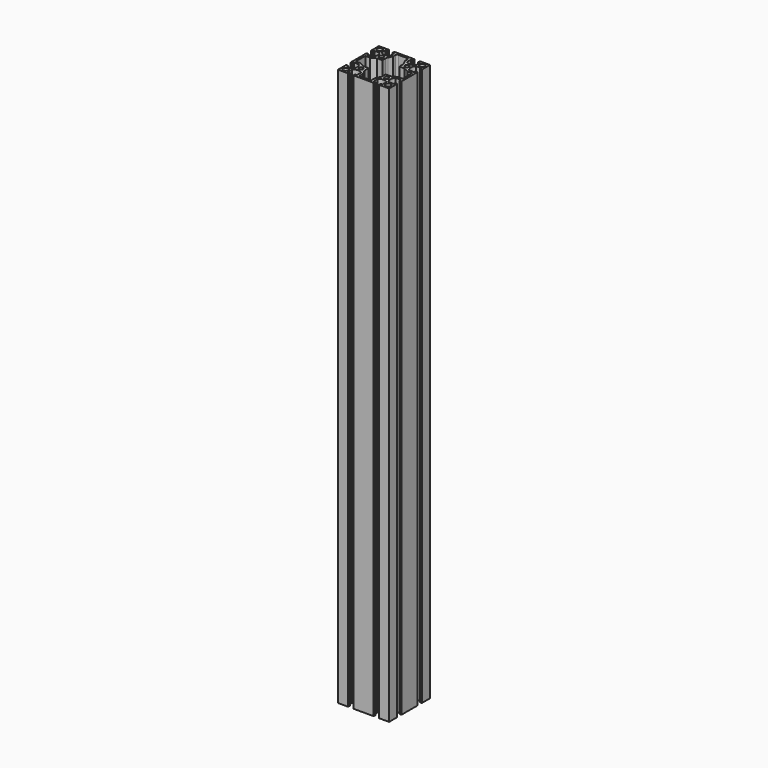
from build123d import *

# Parameters (mm, degrees)
F0_R     = 3
F0_R_2   = 2.5
F1_DEPTH = 655
F2_R     = 2
F3_R     = 7


# Not quite as in the source:
# - a feature names something its author has since deleted; it is built from what else it names


with BuildPart() as f1:
    # F0 (on Top) → F1 (new body)
    with BuildSketch(Plane.XY):
        with BuildLine():
            Line((18.15, -30), (30, -30))
            Line((30, -30), (30, -18.15))
            Line((30, -18.15), (27.5, -18.15))
            Line((27.5, -18.15), (27.5, -20.15))
            Line((27.5, -20.15), (21.5477069044, -20.15))
            ThreePointArc((21.5477069044, -20.15), (19.5, -15), (21.5477069044, -9.85))
            Line((21.5477069044, -9.85), (27.5, -9.85))
            Line((27.5, -9.85), (27.5, -11.85))
            Line((27.5, -11.85), (30, -11.85))
            Line((30, -11.85), (30, 11.85))
            Line((30, 11.85), (27.5, 11.85))
            Line((27.5, 11.85), (27.5, 9.85))
            Line((27.5, 9.85), (21.5477069044, 9.85))
            ThreePointArc((21.5477069044, 9.85), (19.5, 15), (21.5477069044, 20.15))
            Line((21.5477069044, 20.15), (27.5, 20.15))
            Line((27.5, 20.15), (27.5, 18.15))
            Line((27.5, 18.15), (30, 18.15))
            Line((30, 18.15), (30, 30))
            Line((30, 30), (18.15, 30))
            Line((18.15, 30), (18.15, 27.5))
            Line((18.15, 27.5), (20.15, 27.5))
            Line((20.15, 27.5), (20.15, 21.5477069044))
            ThreePointArc((20.15, 21.5477069044), (15, 19.5), (9.85, 21.5477069044))
            Line((9.85, 21.5477069044), (9.85, 27.5))
            Line((9.85, 27.5), (11.85, 27.5))
            Line((11.85, 27.5), (11.85, 30))
            Line((11.85, 30), (-11.85, 30))
            Line((-11.85, 30), (-11.85, 27.5))
            Line((-11.85, 27.5), (-9.85, 27.5))
            Line((-9.85, 27.5), (-9.85, 21.5477069044))
            ThreePointArc((-9.85, 21.5477069044), (-15, 19.5), (-20.15, 21.5477069044))
            Line((-20.15, 21.5477069044), (-20.15, 27.5))
            Line((-20.15, 27.5), (-18.15, 27.5))
            Line((-18.15, 27.5), (-18.15, 30))
            Line((-18.15, 30), (-30, 30))
            Line((-30, 30), (-30, 18.15))
            Line((-30, 18.15), (-27.5, 18.15))
            Line((-27.5, 18.15), (-27.5, 20.15))
            Line((-27.5, 20.15), (-21.5477069044, 20.15))
            ThreePointArc((-21.5477069044, 20.15), (-19.5, 15), (-21.5477069044, 9.85))
            Line((-21.5477069044, 9.85), (-27.5, 9.85))
            Line((-27.5, 9.85), (-27.5, 11.85))
            Line((-27.5, 11.85), (-30, 11.85))
            Line((-30, 11.85), (-30, -11.85))
            Line((-30, -11.85), (-27.5, -11.85))
            Line((-27.5, -11.85), (-27.5, -9.85))
            Line((-27.5, -9.85), (-21.5477069044, -9.85))
            ThreePointArc((-21.5477069044, -9.85), (-19.5, -15), (-21.5477069044, -20.15))
            Line((-21.5477069044, -20.15), (-27.5, -20.15))
            Line((-27.5, -20.15), (-27.5, -18.15))
            Line((-27.5, -18.15), (-30, -18.15))
            Line((-30, -18.15), (-30, -30))
            Line((-30, -30), (-18.15, -30))
            Line((-18.15, -30), (-18.15, -27.5))
            Line((-18.15, -27.5), (-20.15, -27.5))
            Line((-20.15, -27.5), (-20.15, -21.5477069044))
            ThreePointArc((-20.15, -21.5477069044), (-15, -19.5), (-9.85, -21.5477069044))
            Line((-9.85, -21.5477069044), (-9.85, -27.5))
            Line((-9.85, -27.5), (-11.85, -27.5))
            Line((-11.85, -27.5), (-11.85, -30))
            Line((-11.85, -30), (11.85, -30))
            Line((11.85, -30), (11.85, -27.5))
            Line((11.85, -27.5), (9.85, -27.5))
            Line((9.85, -27.5), (9.85, -21.5477069044))
            ThreePointArc((9.85, -21.5477069044), (15, -19.5), (20.15, -21.5477069044))
            Line((20.15, -21.5477069044), (20.15, -27.5))
            Line((20.15, -27.5), (18.15, -27.5))
            Line((18.15, -27.5), (18.15, -30))
        make_face()
        with Locations((-25, -25)):
            Circle(F0_R, mode=Mode.SUBTRACT)
        with Locations((-15, -15)):
            Circle(F0_R_2, mode=Mode.SUBTRACT)
        with Locations((25, -25)):
            Circle(F0_R, mode=Mode.SUBTRACT)
        with Locations((15, -15)):
            Circle(F0_R_2, mode=Mode.SUBTRACT)
        with Locations((-25, 25)):
            Circle(F0_R, mode=Mode.SUBTRACT)
        with Locations((-15, 15)):
            Circle(F0_R_2, mode=Mode.SUBTRACT)
        Polygon((-7, 22), (-7, 27.5), (0, 27.5), (7, 27.5), (7, 22), (10, 16), (10, 10), (16, 10), (22, 7), (27.5, 7), (27.5, 0), (27.5, -7), (22, -7), (16, -10), (10, -10), (10, -16), (7, -22), (7, -27.5), (0, -27.5), (-7, -27.5), (-7, -22), (-10, -16), (-10, -10), (-16, -10), (-22, -7), (-27.5, -7), (-27.5, 0), (-27.5, 7), (-22, 7), (-16, 10), (-10, 10), (-10, 16), align=None, mode=Mode.SUBTRACT)
        with Locations((15, 15)):
            Circle(F0_R_2, mode=Mode.SUBTRACT)
        with Locations((25, 25)):
            Circle(F0_R, mode=Mode.SUBTRACT)
    extrude(amount=F1_DEPTH)

    # F2
    f2_edges = [f1.edges().sort_by_distance(p)[0] for p in [
        (-7, 27.5, 327.5),
        (7, 27.5, 327.5),
    ]]
    fillet(f2_edges, radius=F2_R)

    # F3
    f3_edges = [f1.edges().sort_by_distance(p)[0] for p in [
        (-10, 16, 327.5),
        (10, 16, 327.5),
    ]]
    fillet(f3_edges, radius=F3_R)


solid = f1.part
